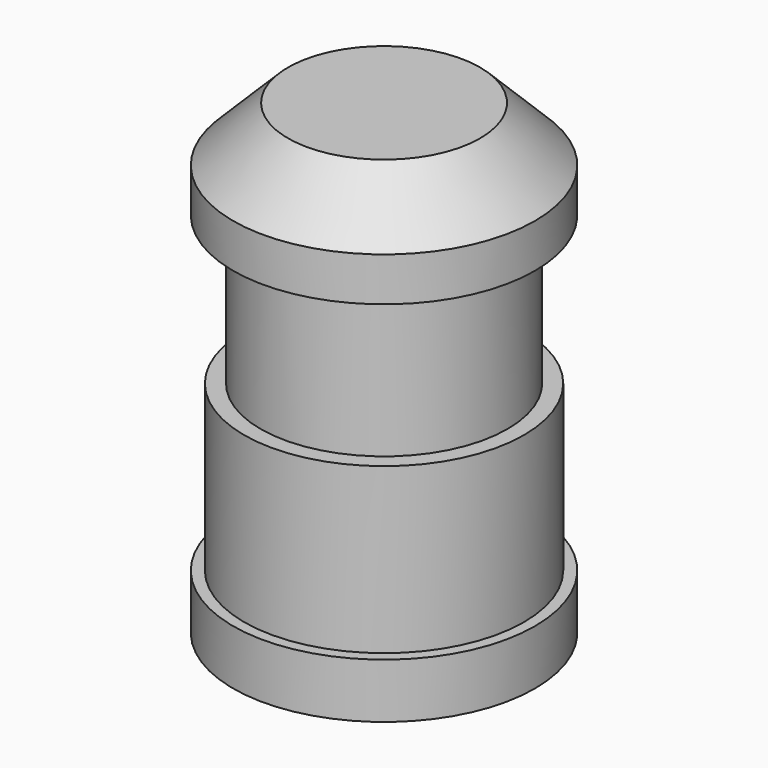
from build123d import *

# Parameters (mm, degrees)
F0_R          = 2.55
F0_R_2        = 2.25
F1_DEPTH      = 4
F2_START      = -3
F0_R_3        = 2.75
F2_DEPTH      = 1
F3_DEPTH      = 4.5
F3_DEPTH_BACK = 1
F4_START      = 2.7
F4_DEPTH      = 1.8
F5_SIZE       = 1


with BuildPart() as f1:
    # F0 (on Top) → F1 (new body)
    with BuildSketch(Plane.XY):
        Circle(F0_R)
        Circle(F0_R_2, mode=Mode.SUBTRACT)
    extrude(amount=-F1_DEPTH)

    # F0 (on Top) → F2 (join)
    with BuildSketch(Plane.XY.offset(F2_START)):
        Circle(F0_R_3)
        Circle(F0_R, mode=Mode.SUBTRACT)
    extrude(amount=-F2_DEPTH)

    # F0 (on Top) → F3 (join, two sides)
    with BuildSketch(Plane.XY) as f3_sk:
        Circle(F0_R_2)
    extrude(amount=F3_DEPTH)
    extrude(f3_sk.sketch, amount=-F3_DEPTH_BACK)

    # F0 (on Top) → F4 (join)
    with BuildSketch(Plane.XY.offset(F4_START)):
        Circle(F0_R_3)
        Circle(F0_R, mode=Mode.SUBTRACT)
        Circle(F0_R)
        Circle(F0_R_2, mode=Mode.SUBTRACT)
    extrude(amount=F4_DEPTH)

    # F5
    f5_edges = [f1.edges().sort_by_distance(p)[0] for p in [
        (-2.75, 0, 4.5),
    ]]
    chamfer(f5_edges, length=F5_SIZE)


solid = f1.part
